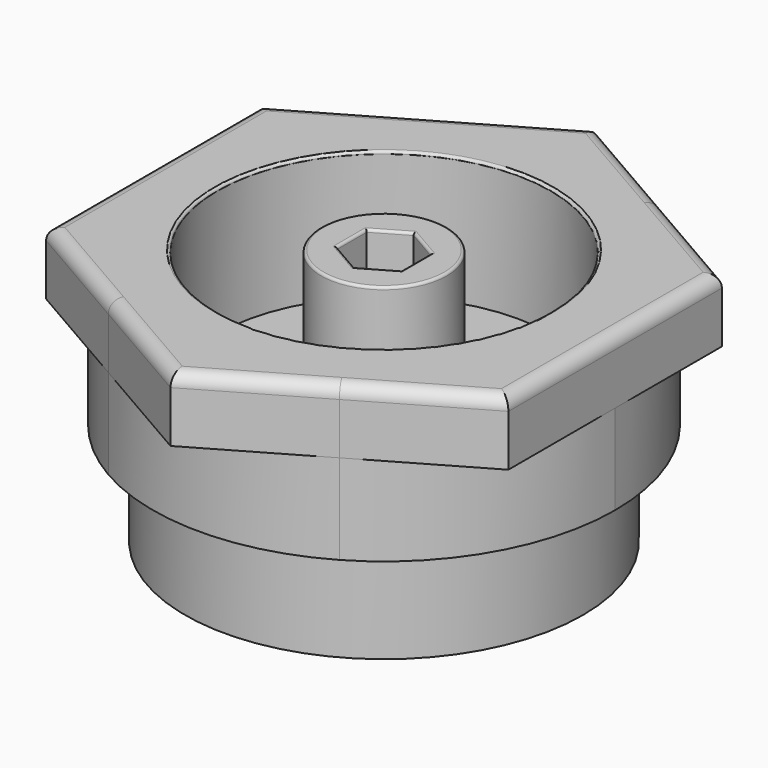
from build123d import *

# Parameters (mm, degrees)
F0_R      = 15.5
F0_R_2    = 13
F1_DEPTH  = 5
F2_R      = 1
F3_DEPTH  = 15
F4_DEPTH  = 5
F5_R      = 4.9
F6_DEPTH  = 10
F8_DEPTH  = 5
F9_R      = 0.2
F10_DEPTH = 7


# Not quite as in the source:
# - a feature names something its author has since deleted; it is built from what else it names


with BuildPart() as f1:
    # F0 (on Top) → F1 (new body)
    with BuildSketch(Plane.XY):
        with BuildLine():
            ThreePointArc((8.9999996925, -15.5884574456), (15.5884571794, -9.0000001537), (18, 0))
            ThreePointArc((18, 0), (15.588457371, 8.9999998218), (9.0000003564, 15.5884570623))
            ThreePointArc((9.0000003564, 15.5884570623), (3.256e-07, 18), (-8.9999997925, 15.5884573879))
            ThreePointArc((-8.9999997925, 15.5884573879), (-15.5884572082, 9.0000001038), (-18, 0))
            ThreePointArc((-18, 0), (-15.588457331, -8.9999998911), (-9.0000002178, -15.5884571424))
            ThreePointArc((-9.0000002178, -15.5884571424), (-3.032e-07, -18), (8.9999996925, -15.5884574456))
        make_face()
        Circle(F0_R, mode=Mode.SUBTRACT)
        with BuildLine():
            ThreePointArc((-8.9999997925, 15.5884573879), (3.256e-07, 18), (9.0000003564, 15.5884570623))
            Line((9.0000003564, 15.5884570623), (0, 20.7846096908))
            Line((0, 20.7846096908), (-8.9999997925, 15.5884573879))
        make_face()
        with BuildLine():
            Line((18, 0), (18, 10.3923048454))
            Line((18, 10.3923048454), (9.0000003564, 15.5884570623))
            ThreePointArc((9.0000003564, 15.5884570623), (15.588457371, 8.9999998218), (18, 0))
        make_face()
        with BuildLine():
            ThreePointArc((-18, 0), (-15.5884572082, 9.0000001038), (-8.9999997925, 15.5884573879))
            Line((-8.9999997925, 15.5884573879), (-18, 10.3923048454))
            Line((-18, 10.3923048454), (-18, 0))
        make_face()
        with BuildLine():
            Line((-18, -10.3923048454), (-9.0000002178, -15.5884571424))
            ThreePointArc((-9.0000002178, -15.5884571424), (-15.588457331, -8.9999998911), (-18, 0))
            Line((-18, 0), (-18, -10.3923048454))
        make_face()
        with BuildLine():
            Line((0, -20.7846096908), (8.9999996925, -15.5884574456))
            ThreePointArc((8.9999996925, -15.5884574456), (-3.032e-07, -18), (-9.0000002178, -15.5884571424))
            Line((-9.0000002178, -15.5884571424), (0, -20.7846096908))
        make_face()
        with BuildLine():
            Line((18, -10.3923048454), (18, 0))
            ThreePointArc((18, 0), (15.5884571794, -9.0000001537), (8.9999996925, -15.5884574456))
            Line((8.9999996925, -15.5884574456), (18, -10.3923048454))
        make_face()
        Circle(F0_R)
        Circle(F0_R_2, mode=Mode.SUBTRACT)
    extrude(amount=F1_DEPTH)

    # F2
    f2_edges = [f1.edges().sort_by_distance(p)[0] for p in [
        (-18, 0, 5),
        (-9, 15.588457, 5),
        (9, 15.588457, 5),
        (18, 0, 5),
        (9, -15.588457, 5),
        (-9, -15.588457, 5),
    ]]
    fillet(f2_edges, radius=F2_R)

    # F0 (on Top) → F3 (join)
    with BuildSketch(Plane.XY):
        Circle(F0_R)
        Circle(F0_R_2, mode=Mode.SUBTRACT)
        Circle(F0_R_2)
    extrude(amount=-F3_DEPTH)

    # F0 (on Top) → F4 (cut)
    with BuildSketch(Plane.XY):
        Circle(F0_R_2)
    extrude(amount=-F4_DEPTH, mode=Mode.SUBTRACT)

    # F5 (on face) → F6 (join, through all)
    with BuildSketch(Plane.XY.offset(-5)):
        Circle(F5_R)
    extrude(amount=F6_DEPTH)

    # F7 (on face) → F8 (cut)
    with BuildSketch(Plane.XY.offset(5)):
        Polygon((-2.5, 1.443375673), (-2.5, -1.443375673), (0, -2.8867513459), (2.5, -1.443375673), (2.5, 1.443375673), (0, 2.8867513459), align=None)
    extrude(amount=-F8_DEPTH, mode=Mode.SUBTRACT)

    # F9
    f9_edges = [f1.edges().sort_by_distance(p)[0] for p in [
        (-4.9, 0, 5),
        (-13, 0, 5),
        (-1.25, 2.165064, 5),
        (1.25, 2.165064, 5),
        (2.5, 0, 5),
        (1.25, -2.165064, 5),
        (-1.25, -2.165064, 5),
        (-2.5, 0, 5),
    ]]
    fillet(f9_edges, radius=F9_R)


with BuildPart() as f10:
    # F0 (on Top) → F10 (new body)
    with BuildSketch(Plane.XY):
        with BuildLine():
            ThreePointArc((8.9999996925, -15.5884574456), (15.5884571794, -9.0000001537), (18, 0))
            ThreePointArc((18, 0), (15.588457371, 8.9999998218), (9.0000003564, 15.5884570623))
            ThreePointArc((9.0000003564, 15.5884570623), (3.256e-07, 18), (-8.9999997925, 15.5884573879))
            ThreePointArc((-8.9999997925, 15.5884573879), (-15.5884572082, 9.0000001038), (-18, 0))
            ThreePointArc((-18, 0), (-15.588457331, -8.9999998911), (-9.0000002178, -15.5884571424))
            ThreePointArc((-9.0000002178, -15.5884571424), (-3.032e-07, -18), (8.9999996925, -15.5884574456))
        make_face()
        Circle(F0_R, mode=Mode.SUBTRACT)
    extrude(amount=-F10_DEPTH)


solid = Compound([f1.part, f10.part])
